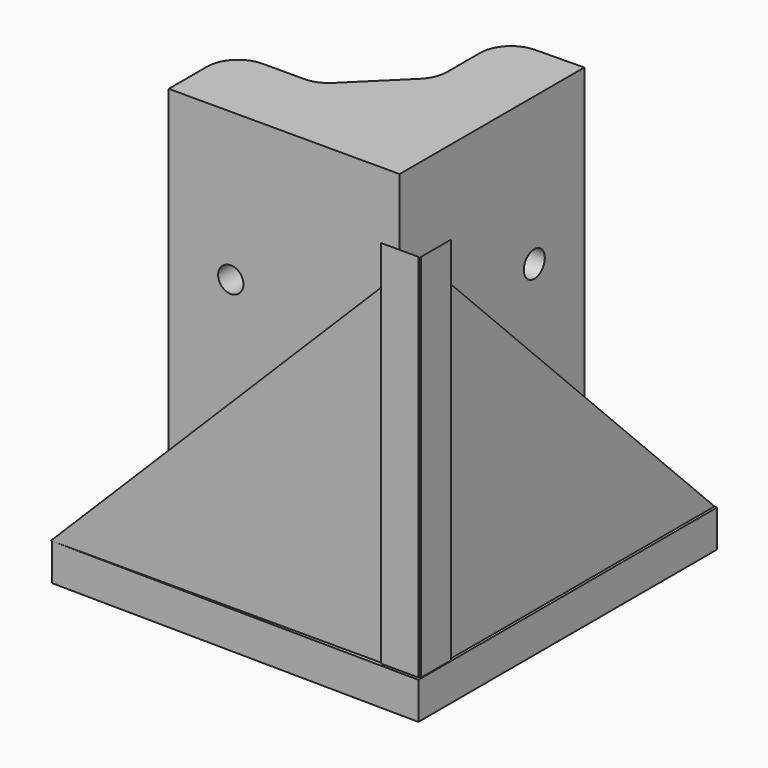
from build123d import *

# Parameters (mm, degrees)
F1_DEPTH       = 7.62
F3_START       = 30.48
F3_DEPTH       = 7.62
F5_DEPTH       = 76.2
F7_DEPTH       = 7.62
F8_R           = 2.6031217073
F9_DEPTH       = 98.806
F10_R          = 2.6995181892
F11_DEPTH      = 47.752
F11_DEPTH_BACK = 45.212
F13_DEPTH      = 1.778


# Not quite as in the source:
# - a feature names something its author has since deleted; it is built from what else it names


with BuildPart() as f1:
    # F0 (on Front) → F1 (new body)
    with BuildSketch(Plane.XZ):
        Polygon((38.4802398158, 76.2), (-37.7197601842, 0), (38.4802398158, 0), align=None)
    extrude(amount=F1_DEPTH)

    # F2 (on Right) → F3 (join)
    with BuildSketch(Plane.YZ.offset(F3_START)):
        Polygon((68.3021095197, 0), (-7.8978904803, 76.2), (-7.8978904803, 0), align=None)
    extrude(amount=F3_DEPTH)


with BuildPart() as f5:
    # F4 (on Top) → F5 (new body)
    with BuildSketch(Plane.XY):
        with BuildLine():
            Line((17.78, 12.7), (17.78, 60.2081210786))
            Line((17.78, 60.2081210786), (7.7990821899, 60.0634692811))
            ThreePointArc((7.7990821899, 60.0634692811), (3.3685570616, 58.1716114676), (1.5411020302, 53.7141360603))
            Line((1.5411020302, 53.7141360603), (1.5411020302, 45.1826832225))
            ThreePointArc((1.5411020302, 45.1826832225), (1.047169173, 42.7272855726), (-0.3577885585, 40.6538726713))
            Line((-0.3577885585, 40.6538726713), (-10.4225503406, 30.7617927566))
            ThreePointArc((-10.4225503406, 30.7617927566), (-12.4690232929, 29.4135101913), (-14.8736597519, 28.9406033078))
            Line((-14.8736597519, 28.9406033078), (-23.3781210786, 28.9406033078))
            ThreePointArc((-23.3781210786, 28.9406033078), (-27.8682491391, 27.0807313683), (-29.7281210786, 22.5906033078))
            Line((-29.7281210786, 22.5906033078), (-29.7281210786, 12.7))
            Line((-29.7281210786, 12.7), (17.78, 12.7))
        make_face()
    extrude(amount=F5_DEPTH)

    # F8 (on Front) → F9 (cut)
    with BuildSketch(Plane.XZ):
        with Locations((-16.9649993712, 45.7831217073)):
            Circle(F8_R)
    extrude(amount=-F9_DEPTH, mode=Mode.SUBTRACT)

    # F10 (on Right) → F11 (cut, two sides)
    with BuildSketch(Plane.YZ) as f11_sk:
        with Locations((47.3486028893, 45.827724101)):
            Circle(F10_R)
    extrude(amount=F11_DEPTH, mode=Mode.SUBTRACT)
    extrude(f11_sk.sketch, amount=-F11_DEPTH_BACK, mode=Mode.SUBTRACT)


with BuildPart() as f7:
    # F6 (on Top) → F7 (new body)
    with BuildSketch(Plane.XY):
        with BuildLine():
            Line((-29.666883871, 22.4884131303), (-29.666883871, 12.7789853141))
            Line((-29.666883871, 12.7789853141), (-37.5426076353, 0))
            Line((-37.5426076353, 0), (-37.5426076353, -7.62))
            Line((-37.5426076353, -7.62), (38.6573923647, -8.5552895431))
            Line((38.6573923647, -8.5552895431), (38.6573923647, 67.6447104569))
            Line((38.6573923647, 67.6447104569), (38.6573923647, 68.276040256))
            Line((38.6573923647, 68.276040256), (30.6627471, 68.276040256))
            Line((30.6627471, 68.276040256), (17.3135716468, 60.3265352547))
            Line((17.3135716468, 60.3265352547), (8.0645363381, 60.3265352547))
            ThreePointArc((8.0645363381, 60.3265352547), (3.5744082776, 58.4666633153), (1.7145363381, 53.9765352547))
            Line((1.7145363381, 53.9765352547), (1.7145363381, 45.4277863735))
            ThreePointArc((1.7145363381, 45.4277863735), (1.2246529933, 42.9820691396), (-0.1694109967, 40.9137113197))
            Line((-0.1694109967, 40.9137113197), (-10.5239810344, 30.6692970018))
            ThreePointArc((-10.5239810344, 30.6692970018), (-12.5811917049, 29.3080014082), (-15.0019310535, 28.8333832011))
            Line((-15.0019310535, 28.8333832011), (-17.6865611632, 28.8384131303))
            Line((-17.6865611632, 28.8384131303), (-23.316883871, 28.8384131303))
            ThreePointArc((-23.316883871, 28.8384131303), (-27.8070119315, 26.9785411909), (-29.666883871, 22.4884131303))
        make_face()
    extrude(amount=-F7_DEPTH)

    # F12 (on face) → F13 (join)
    with BuildSketch(Plane(origin=(0, 0, -7.62), x_dir=(1, 0, 0), z_dir=(0, 0, -1))):
        Polygon((-5.3466960156, -11.8047548458), (-8.1613129005, -11.8047548458), (-8.1613129005, -22.2978685051), (-3.206232097, -27.5444276631), (2.3318054155, -30.6692970018), (8.1613119692, -30.6692970018), (8.1613119692, -25.5040973425), (2.3318054155, -25.5040973425), (-3.206232097, -22.2978685051), (-5.3466960156, -16.7598351836), align=None)
        with BuildLine():
            ThreePointArc((3.9225352044, -15.9396454022), (4.1328254672, -15.1968039625), (4.2037192827, -14.4280325621))
            ThreePointArc((4.2037192827, -14.4280325621), (-3.8316760126, -12.699011237), (2.7814003592, -17.5800268277))
            ThreePointArc((2.7814003592, -17.5800268277), (3.2530804789, -16.6910449513), (3.9225352044, -15.9396454022))
        make_face()
        with BuildLine():
            ThreePointArc((3.9225352044, -15.9396454022), (3.2530804789, -16.6910449513), (2.7814003592, -17.5800268277))
            ThreePointArc((2.7814003592, -17.5800268277), (3.4508550847, -16.8286272786), (3.9225352044, -15.9396454022))
        make_face()
        with BuildLine():
            ThreePointArc((3.9225352044, -15.9396454022), (3.4508550847, -16.8286272786), (2.7814003592, -17.5800268277))
            ThreePointArc((2.7814003592, -17.5800268277), (5.9351641632, -23.2244651349), (10.9076548463, -19.0916396677))
            ThreePointArc((10.9076548463, -19.0916396677), (8.4329568887, -15.2599636552), (3.9225352044, -15.9396454022))
        make_face()
    extrude(amount=F13_DEPTH)


solid = Compound([f1.part, f5.part, f7.part])
